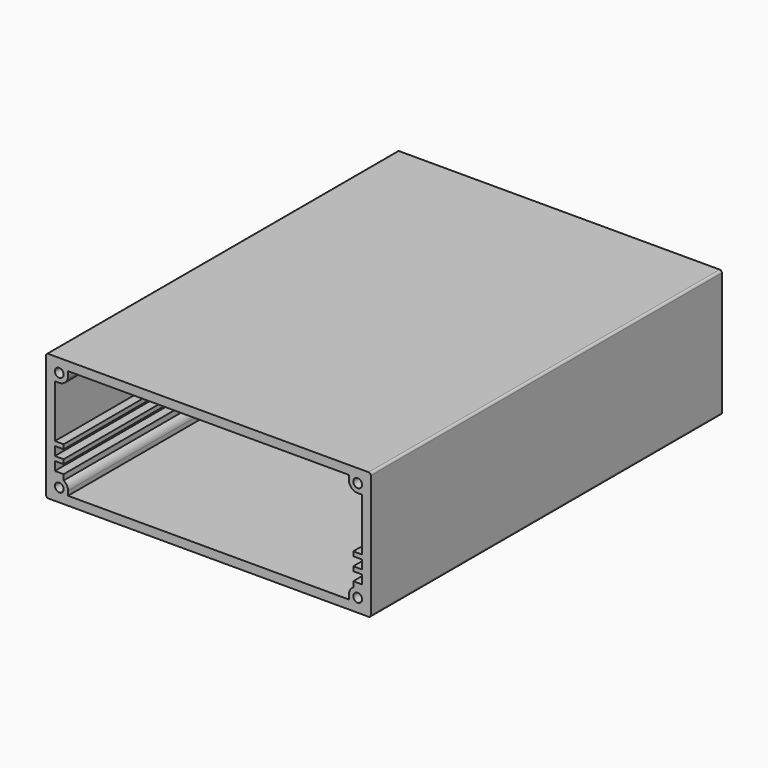
from build123d import *

# Parameters (mm, degrees)
F0_W     = 2
F0_H     = 1
F1_DEPTH = 100


with BuildPart() as f1:
    # F0 (on Front) → F1 (new body)
    with BuildSketch(Plane.XZ):
        with BuildLine():
            Line((37.4444444444, 14.6527777778), (-35.5555555556, 14.6527777778))
            ThreePointArc((-35.5555555556, 14.6527777778), (-35.9091089461, 14.5063311684), (-36.0555555556, 14.1527777778))
            Line((-36.0555555556, 14.1527777778), (-36.0555555556, -13.8472222222))
            ThreePointArc((-36.0555555556, -13.8472222222), (-35.9091089461, -14.2007756128), (-35.5555555556, -14.3472222222))
            Line((-35.5555555556, -14.3472222222), (37.4444444444, -14.3472222222))
            ThreePointArc((37.4444444444, -14.3472222222), (37.797997835, -14.2007756128), (37.9444444444, -13.8472222222))
            Line((37.9444444444, -13.8472222222), (37.9444444444, 14.1527777778))
            ThreePointArc((37.9444444444, 14.1527777778), (37.797997835, 14.5063311684), (37.4444444444, 14.6527777778))
        make_face()
        Polygon((-31.0555555556, 12.6527777778), (32.9444444444, 12.6527777778), (34.9444444444, 12.6527777778), (35.9444444444, 12.6527777778), (35.9444444444, 11.6527777778), (35.9444444444, 9.6527777778), (35.9444444444, -2.3472222222), (35.9444444444, -3.3472222222), (35.9444444444, -5.3472222222), (35.9444444444, -6.3472222222), (35.9444444444, -8.3472222222), (35.9444444444, -9.3472222222), (35.9444444444, -11.3472222222), (35.9444444444, -12.3472222222), (34.9444444444, -12.3472222222), (32.9444444444, -12.3472222222), (-31.0555555556, -12.3472222222), (-33.0555555556, -12.3472222222), (-34.0555555556, -12.3472222222), (-34.0555555556, -11.3472222222), (-34.0555555556, -9.3472222222), (-34.0555555556, -8.3472222222), (-34.0555555556, -6.3472222222), (-34.0555555556, -5.3472222222), (-34.0555555556, -3.3472222222), (-34.0555555556, -2.3472222222), (-34.0555555556, 9.6527777778), (-34.0555555556, 11.6527777778), (-34.0555555556, 12.6527777778), (-33.0555555206, 12.6527777778), align=None, mode=Mode.SUBTRACT)
        with BuildLine():
            Line((34.9444444444, 12.6527777778), (32.9444444444, 12.6527777778))
            Line((32.9444444444, 12.6527777778), (32.9444444444, 11.6527777778))
            ThreePointArc((32.9444444444, 11.6527777778), (33.5302308821, 10.2385642154), (34.9444444444, 9.6527777778))
            Line((34.9444444444, 9.6527777778), (35.9444444444, 9.6527777778))
            Line((35.9444444444, 9.6527777778), (35.9444444444, 11.6527777778))
            ThreePointArc((35.9444444444, 11.6527777778), (34.2373376633, 10.9456709966), (34.9444444444, 12.6527777778))
        make_face()
        with BuildLine():
            Line((35.9444444444, -11.3472222222), (35.9444444444, -9.3472222222))
            Line((35.9444444444, -9.3472222222), (34.9444444444, -9.3472222222))
            ThreePointArc((34.9444444444, -9.3472222222), (34.4268063542, -9.4153705696), (33.9444444444, -9.6151714147))
            ThreePointArc((33.9444444444, -9.6151714147), (33.2123936369, -10.3472222222), (32.9444444444, -11.3472222222))
            Line((32.9444444444, -11.3472222222), (32.9444444444, -12.3472222222))
            Line((32.9444444444, -12.3472222222), (34.9444444444, -12.3472222222))
            ThreePointArc((34.9444444444, -12.3472222222), (34.2373376633, -10.640115441), (35.9444444444, -11.3472222222))
        make_face()
        with BuildLine():
            Line((-31.0555555556, 11.6527777778), (-31.0555555556, 12.6527777778))
            Line((-31.0555555556, 12.6527777778), (-33.0555555206, 12.6527777778))
            ThreePointArc((-33.0555555206, 12.6527777778), (-32.348448762, 12.3598845466), (-32.0555555556, 11.6527777778))
            ThreePointArc((-32.0555555556, 11.6527777778), (-33.0555555556, 10.6527777778), (-34.0555555556, 11.6527777778))
            Line((-34.0555555556, 11.6527777778), (-34.0555555556, 9.6527777778))
            Line((-34.0555555556, 9.6527777778), (-33.0555555556, 9.6527777778))
            ThreePointArc((-33.0555555556, 9.6527777778), (-31.6413419932, 10.2385642154), (-31.0555555556, 11.6527777778))
        make_face()
        with BuildLine():
            Line((-33.0555555556, -9.3472222222), (-34.0555555556, -9.3472222222))
            Line((-34.0555555556, -9.3472222222), (-34.0555555556, -11.3472222222))
            ThreePointArc((-34.0555555556, -11.3472222222), (-33.0555555556, -10.3472222222), (-32.0555555556, -11.3472222222))
            ThreePointArc((-32.0555555556, -11.3472222222), (-32.3484487744, -12.0543290034), (-33.0555555556, -12.3472222222))
            Line((-33.0555555556, -12.3472222222), (-31.0555555556, -12.3472222222))
            Line((-31.0555555556, -12.3472222222), (-31.0555555556, -11.3472222222))
            ThreePointArc((-31.0555555556, -11.3472222222), (-31.323504748, -10.3472222222), (-32.0555555556, -9.6151714147))
            ThreePointArc((-32.0555555556, -9.6151714147), (-32.5379174654, -9.4153705696), (-33.0555555556, -9.3472222222))
        make_face()
        with BuildLine():
            Line((35.9444444444, -9.3472222222), (35.9444444444, -8.3472222222))
            Line((35.9444444444, -8.3472222222), (33.9444444444, -8.3472222222))
            Line((33.9444444444, -8.3472222222), (33.9444444444, -9.6151714147))
            ThreePointArc((33.9444444444, -9.6151714147), (34.4268063542, -9.4153705696), (34.9444444444, -9.3472222222))
            Line((34.9444444444, -9.3472222222), (35.9444444444, -9.3472222222))
        make_face()
        with BuildLine():
            Line((-32.0555555556, -8.3472222222), (-34.0555555556, -8.3472222222))
            Line((-34.0555555556, -8.3472222222), (-34.0555555556, -9.3472222222))
            Line((-34.0555555556, -9.3472222222), (-33.0555555556, -9.3472222222))
            ThreePointArc((-33.0555555556, -9.3472222222), (-32.5379174654, -9.4153705696), (-32.0555555556, -9.6151714147))
            Line((-32.0555555556, -9.6151714147), (-32.0555555556, -8.3472222222))
        make_face()
        with Locations((34.9444444444, -5.8472222222)):
            Rectangle(F0_W, F0_H)
        with Locations((-33.0555555556, -5.8472222222)):
            Rectangle(F0_W, F0_H)
        with Locations((-33.0555555556, -2.8472222222)):
            Rectangle(F0_W, F0_H)
        with Locations((34.9444444444, -2.8472222222)):
            Rectangle(F0_W, F0_H)
        with BuildLine():
            Line((35.9444444444, 12.6527777778), (34.9444444444, 12.6527777778))
            ThreePointArc((34.9444444444, 12.6527777778), (35.6515512256, 12.359884559), (35.9444444444, 11.6527777778))
            Line((35.9444444444, 11.6527777778), (35.9444444444, 12.6527777778))
        make_face()
        with BuildLine():
            Line((35.9444444444, -12.3472222222), (35.9444444444, -11.3472222222))
            ThreePointArc((35.9444444444, -11.3472222222), (35.6515512256, -12.0543290034), (34.9444444444, -12.3472222222))
            Line((34.9444444444, -12.3472222222), (35.9444444444, -12.3472222222))
        make_face()
        with BuildLine():
            ThreePointArc((-34.0555555556, 11.6527777778), (-33.7626623244, 12.3598845713), (-33.0555555206, 12.6527777778))
            Line((-33.0555555206, 12.6527777778), (-34.0555555556, 12.6527777778))
            Line((-34.0555555556, 12.6527777778), (-34.0555555556, 11.6527777778))
        make_face()
        with BuildLine():
            ThreePointArc((-33.0555555556, -12.3472222222), (-33.7626623367, -12.0543290034), (-34.0555555556, -11.3472222222))
            Line((-34.0555555556, -11.3472222222), (-34.0555555556, -12.3472222222))
            Line((-34.0555555556, -12.3472222222), (-33.0555555556, -12.3472222222))
        make_face()
    extrude(amount=F1_DEPTH)


solid = f1.part
